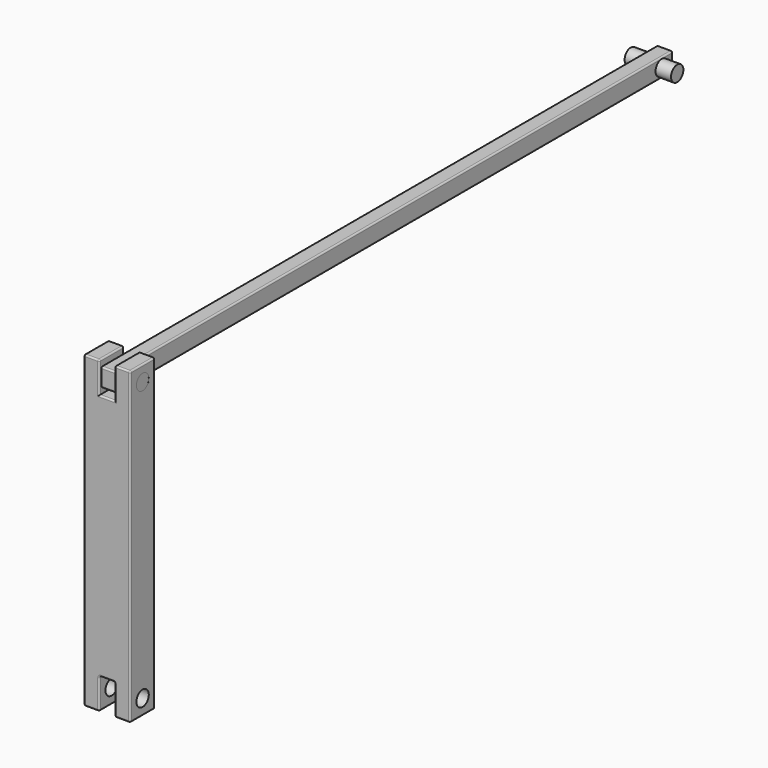
from build123d import *

# Parameters (mm, degrees)
F1_DEPTH      = 20
F3_D          = 10
F4_R          = 1
F5_W          = 450
F5_H          = 12
F5_R          = 5
F6_DEPTH      = 10
F7_R          = 0.99999
F8_DEPTH      = 20
F8_DEPTH_BACK = 10


# Not quite as in the source:
# - a fillet or chamfer is up to 0.001 mm smaller than in the source, because OpenCascade refuses the exact size


with BuildPart() as f1:
    # F0 (on Front) → F1 (new body)
    with BuildSketch(Plane.XZ):
        Polygon((10, 100), (0, 100), (0, 0), (0, -100), (10, -100), (10, -80), (20, -80), (20, -100), (30, -100), (30, 0), (30, 100), (20, 100), (20, 80), (10, 80), align=None)
    extrude(amount=F1_DEPTH)

    # F3 (through all)
    with Locations(Plane(origin=(0, 0, 0), x_dir=(0, 1, 0), z_dir=(-1, 0, 0))):
        with Locations((-10, -90), (-10, 90)):
            Hole(F3_D / 2)

    # F4
    f4_edges = [f1.edges().sort_by_distance(p)[0] for p in [
        (5, 0, 100),
        (0, 0, 0),
        (5, 0, -100),
        (10, 0, -90),
        (15, 0, -80),
        (20, 0, -90),
        (25, 0, -100),
        (30, 0, 0),
        (25, 0, 100),
        (20, 0, 90),
        (15, 0, 80),
        (10, 0, 90),
        (30, -20, 0),
        (5, -20, 100),
        (0, -20, 0),
        (5, -20, -100),
        (10, -20, -90),
        (15, -20, -80),
        (20, -20, -90),
        (25, -20, -100),
        (25, -20, 100),
        (20, -20, 90),
        (15, -20, 80),
        (10, -20, 90),
        (30, -10, 100),
        (20, -10, 100),
        (10, -10, 100),
        (0, -10, 100),
        (20, -10, -100),
        (30, -10, -100),
        (0, -10, -100),
        (10, -10, -100),
        (10, -10, -80),
        (20, -10, -80),
    ]]
    fillet(f4_edges, radius=F4_R)


with BuildPart() as f6:
    # F5 (on face) → F6 (new body, through all)
    with BuildSketch(Plane.YZ.offset(10)):
        with Locations((206, 90)):
            Rectangle(F5_W, F5_H)
        with Locations((-10, 90)):
            Circle(F5_R, mode=Mode.SUBTRACT)
        with Locations((422, 90)):
            Circle(F5_R, mode=Mode.SUBTRACT)
    extrude(amount=F6_DEPTH)

    # F7 (radius 1 in the source; OpenCascade refuses exactly that, so slightly less here)
    f7_edges = [f6.edges().sort_by_distance(p)[0] for p in [
        (15, 431, 96),
        (15, -19, 96),
        (10, 206, 96),
        (20, 206, 96),
        (15, 431, 84),
        (10, 431, 90),
        (20, 431, 90),
        (15, -19, 84),
        (10, 206, 84),
        (20, 206, 84),
        (10, -19, 90),
        (20, -19, 90),
    ]]
    fillet(f7_edges, radius=F7_R)

    # F5 (on face) → F8 (join, two sides)
    with BuildSketch(Plane.YZ.offset(10)) as f8_sk:
        with Locations((-10, 90)):
            Circle(F5_R)
        with Locations((422, 90)):
            Circle(F5_R)
    extrude(amount=F8_DEPTH)
    extrude(f8_sk.sketch, amount=-F8_DEPTH_BACK)


solid = Compound([f1.part, f6.part])
